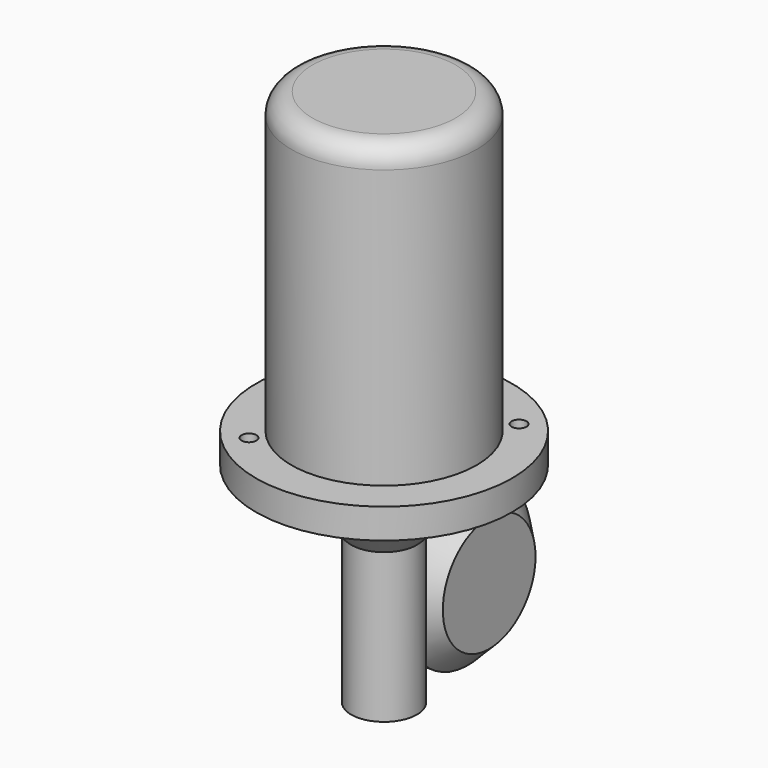
from build123d import *

# Parameters (mm, degrees)
F0_R          = 31
F0_R_2        = 11.0794827648
F1_DEPTH      = 100
F2_R          = 7
F0_R_3        = 42.8779340108
F0_R_4        = 2.5
F3_DEPTH      = 10
F4_DEPTH      = 30
F5_DEPTH      = 30
F6_SIZE       = 19.99999
F7_DEPTH      = 50
F8_R          = 26.3926129655
F9_DEPTH      = 12.5
F10_S5_R      = 11.00001
F10_T6_DEPTH  = 39
F10_S11_R     = 11.00001
F10_T12_DEPTH = 39


# Not quite as in the source:
# - a fillet or chamfer that OpenCascade refuses, or shapes differently, is made with other operations: its cross-section is extruded or revolved along the edge and cut away or added
# - a fillet or chamfer is up to 0.001 mm smaller than in the source, because OpenCascade refuses the exact size


with BuildPart() as f1:
    # F0 (on Top) → F1 (new body)
    with BuildSketch(Plane.XY):
        Circle(F0_R)
        Circle(F0_R_2, mode=Mode.SUBTRACT)
        Circle(F0_R_2)
    extrude(amount=F1_DEPTH)

    # F2
    f2_edges = [f1.edges().sort_by_distance(p)[0] for p in [
        (-31, 0, 100),
    ]]
    fillet(f2_edges, radius=F2_R)

    # F0 (on Top) → F3 (join)
    with BuildSketch(Plane.XY):
        Circle(F0_R_3)
        with Locations((-25.1022907321, -25.1022907321)):
            Circle(F0_R_4, mode=Mode.SUBTRACT)
        Circle(F0_R, mode=Mode.SUBTRACT)
        with Locations((25.1022907321, 25.1022907321)):
            Circle(F0_R_4, mode=Mode.SUBTRACT)
    extrude(amount=-F3_DEPTH)

    # F0 (on Top) → F4 (join)
    with BuildSketch(Plane.XY):
        Circle(F0_R_2)
    extrude(amount=-F4_DEPTH)

    # F0 (on Top) → F5 (join)
    with BuildSketch(Plane.XY):
        Circle(F0_R)
        Circle(F0_R_2, mode=Mode.SUBTRACT)
    extrude(amount=-F5_DEPTH)

    # F6 (size 20 in the source; OpenCascade refuses exactly that, so slightly less here)
    f6_edges = [f1.edges().sort_by_distance(p)[0] for p in [
        (-31, 0, -30),
    ]]
    chamfer(f6_edges, length=F6_SIZE)

    # F7 (add): a face of the model
    f7_faces = [f1.faces().sort_by_distance(p)[0] for p in [
        (0, 0, -30),
    ]]
    extrude(f7_faces, amount=F7_DEPTH)

    # F8 (on Right) → F9 (join, symmetric)
    with BuildSketch(Plane.YZ):
        with Locations((28.3597782254, -52.3124225438)):
            Circle(F8_R)
    extrude(amount=F9_DEPTH, both=True)

    # F10: chamfer of 7 on 2 edges, made by hand


with BuildPart() as f10_tool2:
    # F10_s3 → F10_t4 (revolve)
    with BuildSketch(Plane.XY.offset(-52.3124225438)):
        Polygon((5.5, 54.7523911909), (12.5, 47.7523911909), (12.5, 54.7523911909), align=None)
    revolve(axis=Axis((12.5, 28.3597782254, -52.3124225438), (1, 0, 0)))

    # F10_s5 → F10_t6 (cut, symmetric)
    with BuildSketch(Plane.XY.offset(-52.3)):
        Circle(F10_S5_R)
    extrude(amount=F10_T6_DEPTH, both=True, mode=Mode.SUBTRACT)


with BuildPart() as f1_1:
    add(f1.part)

    # F10_t1: cut F10_tool2
    add(f10_tool2.part, mode=Mode.SUBTRACT)


with BuildPart() as f10_tool8:
    # F10_s9 → F10_t10 (revolve)
    with BuildSketch(Plane.XY.offset(-52.3124225438)):
        Polygon((-5.5, 54.7523911909), (-12.5, 47.7523911909), (-12.5, 54.7523911909), align=None)
    revolve(axis=Axis((-12.5, 28.3597782254, -52.3124225438), (1, 0, 0)))

    # F10_s11 → F10_t12 (cut, symmetric)
    with BuildSketch(Plane.XY.offset(-52.3)):
        Circle(F10_S11_R)
    extrude(amount=F10_T12_DEPTH, both=True, mode=Mode.SUBTRACT)


with BuildPart() as f1_2:
    add(f1_1.part)

    # F10_t7: cut F10_tool8
    add(f10_tool8.part, mode=Mode.SUBTRACT)


solid = f1_2.part
